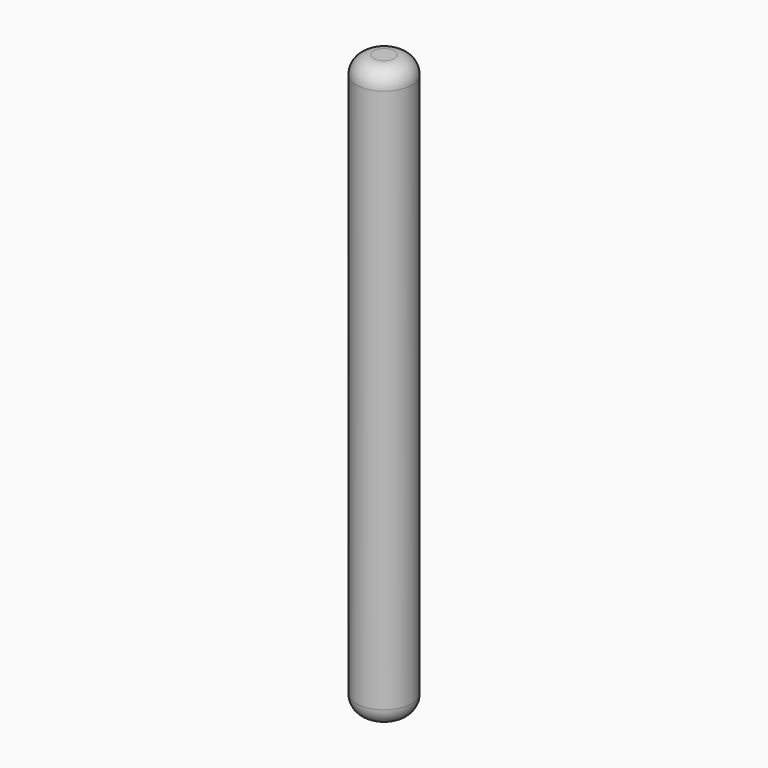
from build123d import *

# Parameters (mm, degrees)
F1_R     = 1.5875
F2_DEPTH = 33
F3_R     = 1


with BuildPart() as f2:
    # F1 (on Top) → F2 (new body)
    with BuildSketch(Plane.XY):
        Circle(F1_R)
    extrude(amount=F2_DEPTH)

    # F3
    f3_edges = [f2.edges().sort_by_distance(p)[0] for p in [
        (-1.5875, 0, 33),
        (-1.5875, 0, 0),
    ]]
    fillet(f3_edges, radius=F3_R)


solid = f2.part
